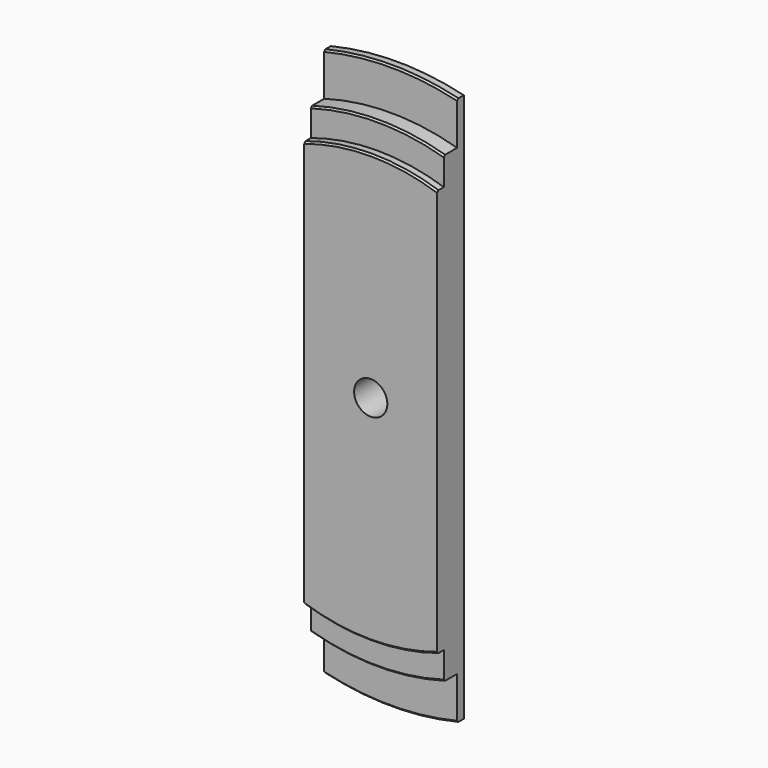
from build123d import *

# Parameters (mm, degrees)
F1_DEPTH = 5
F2_DEPTH = 15
F0_R     = 10
F3_DEPTH = 20
F4_DEPTH = 30
F5_SIZE  = 1


with BuildPart() as f1:
    # F0 (on Front) → F1 (new body)
    with BuildSketch(Plane.XZ):
        with BuildLine():
            Line((40, 139.3735986477), (40, 165.2271164186))
            ThreePointArc((40, 165.2271164186), (0, 170), (-40, 165.2271164186))
            Line((-40, 165.2271164186), (-40, 139.3735986477))
            ThreePointArc((-40, 139.3735986477), (0, 145), (40, 139.3735986477))
        make_face()
        with BuildLine():
            Line((-40, 139.3735986477), (-40, 165.2271164186))
            ThreePointArc((-40, 165.2271164186), (-170, 0), (-40, -165.2271164186))
            Line((-40, -165.2271164186), (-40, -139.3735986477))
            ThreePointArc((-40, -139.3735986477), (-145, 0), (-40, 139.3735986477))
        make_face()
        with BuildLine():
            ThreePointArc((-40, -165.2271164186), (0, -170), (40, -165.2271164186))
            Line((40, -165.2271164186), (40, -139.3735986477))
            ThreePointArc((40, -139.3735986477), (0, -145), (-40, -139.3735986477))
            Line((-40, -139.3735986477), (-40, -165.2271164186))
        make_face()
        with BuildLine():
            ThreePointArc((40, -165.2271164186), (133.6038921589, -105.1189802081), (170, 0))
            ThreePointArc((170, 0), (133.6038921589, 105.1189802081), (40, 165.2271164186))
            Line((40, 165.2271164186), (40, 139.3735986477))
            ThreePointArc((40, 139.3735986477), (115.812348219, 87.2496418331), (145, 0))
            ThreePointArc((145, 0), (115.812348219, -87.2496418331), (40, -139.3735986477))
            Line((40, -139.3735986477), (40, -165.2271164186))
        make_face()
    extrude(amount=F1_DEPTH)

    # F0 (on Front) → F2 (join)
    with BuildSketch(Plane.XZ):
        with BuildLine():
            Line((40, 122.6417547167), (40, 139.3735986477))
            ThreePointArc((40, 139.3735986477), (0, 145), (-40, 139.3735986477))
            Line((-40, 139.3735986477), (-40, 122.6417547167))
            ThreePointArc((-40, 122.6417547167), (0, 129), (40, 122.6417547167))
        make_face()
        with BuildLine():
            Line((-40, 122.6417547167), (-40, 139.3735986477))
            ThreePointArc((-40, 139.3735986477), (-145, 0), (-40, -139.3735986477))
            Line((-40, -139.3735986477), (-40, -122.6417547167))
            ThreePointArc((-40, -122.6417547167), (-129, 0), (-40, 122.6417547167))
        make_face()
        with BuildLine():
            ThreePointArc((-40, -139.3735986477), (0, -145), (40, -139.3735986477))
            Line((40, -139.3735986477), (40, -122.6417547167))
            ThreePointArc((40, -122.6417547167), (0, -129), (-40, -122.6417547167))
            Line((-40, -122.6417547167), (-40, -139.3735986477))
        make_face()
        with BuildLine():
            ThreePointArc((145, 0), (115.812348219, 87.2496418331), (40, 139.3735986477))
            Line((40, 139.3735986477), (40, 122.6417547167))
            ThreePointArc((40, 122.6417547167), (104.4054596274, 75.7660874006), (129, 0))
            ThreePointArc((129, 0), (104.4054596274, -75.7660874006), (40, -122.6417547167))
            Line((40, -122.6417547167), (40, -139.3735986477))
            ThreePointArc((40, -139.3735986477), (115.812348219, -87.2496418331), (145, 0))
        make_face()
    extrude(amount=F2_DEPTH)

    # F0 (on Front) → F3 (join)
    with BuildSketch(Plane.XZ):
        with BuildLine():
            Line((40, -122.6417547167), (40, 122.6417547167))
            ThreePointArc((40, 122.6417547167), (0, 129), (-40, 122.6417547167))
            Line((-40, 122.6417547167), (-40, -122.6417547167))
            ThreePointArc((-40, -122.6417547167), (0, -129), (40, -122.6417547167))
        make_face()
        Circle(F0_R, mode=Mode.SUBTRACT)
    extrude(amount=F3_DEPTH)

    # F0 (on Front) → F4 (cut)
    with BuildSketch(Plane.XZ):
        with BuildLine():
            ThreePointArc((40, -165.2271164186), (133.6038921589, -105.1189802081), (170, 0))
            ThreePointArc((170, 0), (133.6038921589, 105.1189802081), (40, 165.2271164186))
            Line((40, 165.2271164186), (40, 139.3735986477))
            ThreePointArc((40, 139.3735986477), (115.812348219, 87.2496418331), (145, 0))
            ThreePointArc((145, 0), (115.812348219, -87.2496418331), (40, -139.3735986477))
            Line((40, -139.3735986477), (40, -165.2271164186))
        make_face()
        with BuildLine():
            Line((-40, 139.3735986477), (-40, 165.2271164186))
            ThreePointArc((-40, 165.2271164186), (-170, 0), (-40, -165.2271164186))
            Line((-40, -165.2271164186), (-40, -139.3735986477))
            ThreePointArc((-40, -139.3735986477), (-145, 0), (-40, 139.3735986477))
        make_face()
        with BuildLine():
            ThreePointArc((145, 0), (115.812348219, 87.2496418331), (40, 139.3735986477))
            Line((40, 139.3735986477), (40, 122.6417547167))
            ThreePointArc((40, 122.6417547167), (104.4054596274, 75.7660874006), (129, 0))
            ThreePointArc((129, 0), (104.4054596274, -75.7660874006), (40, -122.6417547167))
            Line((40, -122.6417547167), (40, -139.3735986477))
            ThreePointArc((40, -139.3735986477), (115.812348219, -87.2496418331), (145, 0))
        make_face()
        with BuildLine():
            Line((-40, 122.6417547167), (-40, 139.3735986477))
            ThreePointArc((-40, 139.3735986477), (-145, 0), (-40, -139.3735986477))
            Line((-40, -139.3735986477), (-40, -122.6417547167))
            ThreePointArc((-40, -122.6417547167), (-129, 0), (-40, 122.6417547167))
        make_face()
        with BuildLine():
            ThreePointArc((129, 0), (104.4054596274, 75.7660874006), (40, 122.6417547167))
            Line((40, 122.6417547167), (40, -122.6417547167))
            ThreePointArc((40, -122.6417547167), (104.4054596274, -75.7660874006), (129, 0))
        make_face()
    extrude(amount=F4_DEPTH, mode=Mode.SUBTRACT)

    # F5
    f5_edges = [f1.edges().sort_by_distance(p)[0] for p in [
        (0, -20, -129),
        (0, -15, -145),
        (0, -15, 145),
        (0, -5, 170),
        (0, -5, -170),
        (0, -20, 129),
    ]]
    chamfer(f5_edges, length=F5_SIZE)


solid = f1.part
